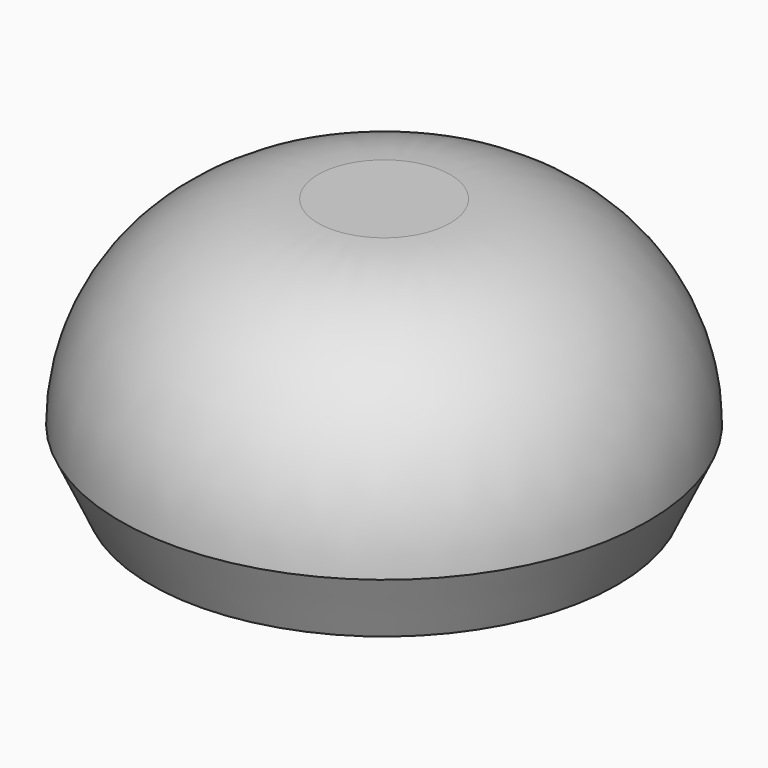
from build123d import *

# Parameters (mm, degrees)
F0_W     = 25.4
F0_H     = 25.4
F2_R     = 19.05
F3_SIZE2 = 2.961044
F3_SIZE  = 6.34999


# Not quite as in the source:
# - a fillet or chamfer is up to 0.001 mm smaller than in the source, because OpenCascade refuses the exact size


with BuildPart() as f1:
    # F0 (on Front) → F1 (revolve)
    with BuildSketch(Plane.XZ):
        with Locations((12.7, 12.7)):
            Rectangle(F0_W, F0_H)
    revolve(axis=Axis((0, 0, 12.7), (0, 0, 1)))

    # F2
    f2_edges = [f1.edges().sort_by_distance(p)[0] for p in [
        (-25.4, 0, 25.4),
    ]]
    fillet(f2_edges, radius=F2_R)

    # F3 (size 6.35 and 2.9610536293 in the source; OpenCascade refuses exactly that, so slightly less here)
    f3_edges = [f1.edges().sort_by_distance(p)[0] for p in [
        (-25.4, 0, 0),
    ]]
    chamfer(f3_edges, length=F3_SIZE, length2=F3_SIZE2)


solid = f1.part
